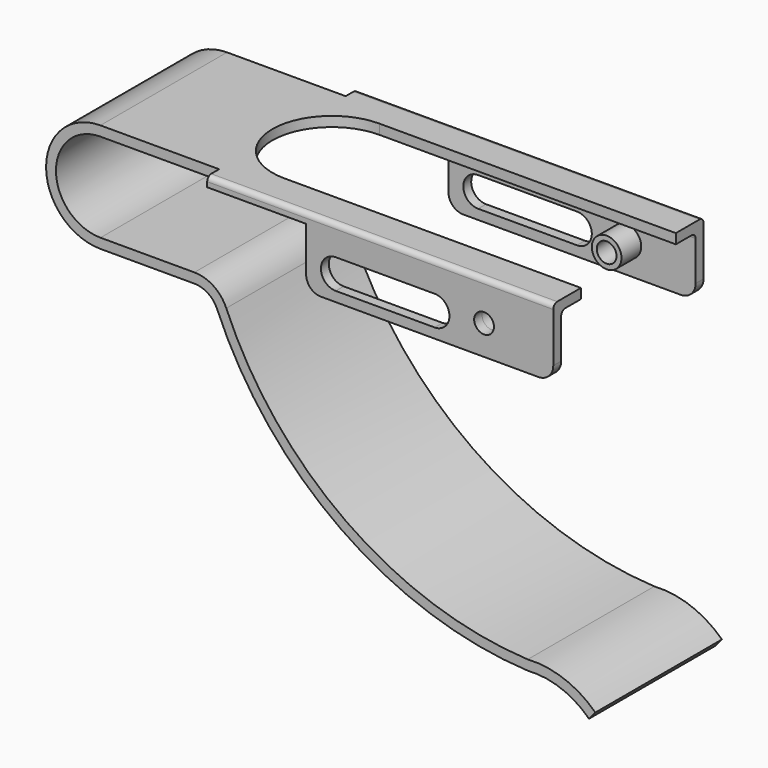
from build123d import *

# Parameters (mm, degrees)
F1_DEPTH  = 16
F2_W      = 70
F2_H      = 3
F3_DEPTH  = 2
F4_W      = 50
F4_H      = 12
F5_DEPTH  = 2
F6_R      = 1
F9_DEPTH  = 2
F11_DEPTH = 38.001
F13_D     = 4
F14_R     = 3
F14_R_2   = 2
F15_DEPTH = 5
F16_R     = 3


# Not quite as in the source:
# - a pattern or mirror of a feature is missing from the dataset's text; its kind, count and spacing are read off the source's solid


with BuildPart() as f1:
    # F0 (on Front) → F1 (new body)
    with BuildSketch(Plane.XZ):
        with BuildLine():
            Line((94, 11), (0, 11))
            ThreePointArc((0, 11), (-11, 0), (0, -11))
            Line((0, -11), (19, -11))
            ThreePointArc((19, -11), (21.7648271935, -11.8339790459), (23.607331209, -14.0577077639))
            ThreePointArc((23.607331209, -14.0577077639), (48.6917034204, -45.0930519948), (86.4506679072, -58.0034711071))
            ThreePointArc((86.4506679072, -58.0034711071), (93.1291053538, -58.9355091014), (98.8304523125, -62.5361846502))
            Line((98.8304523125, -62.5361846502), (100.1194642859, -61))
            ThreePointArc((100.1194642859, -61), (93.803453137, -57.0525770858), (86.4301074938, -56))
            ThreePointArc((86.4301074938, -56), (49.7895156694, -43.4202136678), (25.4502636926, -13.2807908695))
            ThreePointArc((25.4502636926, -13.2807908695), (22.8707580709, -10.1675706642), (19, -9))
            Line((19, -9), (0, -9))
            ThreePointArc((0, -9), (-9, 0), (0, 9))
            Line((0, 9), (94, 9))
            Line((94, 9), (94, 11))
        make_face()
    extrude(amount=F1_DEPTH)

    # F2 (on face) → F3 (join)
    with BuildSketch(Plane.XY.offset(11)):
        with Locations((59, -17.5)):
            Rectangle(F2_W, F2_H)
    extrude(amount=-F3_DEPTH)

    # F4 (on face) → F5 (join)
    with BuildSketch(Plane.XZ.offset(19)):
        with Locations((69, 3)):
            Rectangle(F4_W, F4_H)
    extrude(amount=-F5_DEPTH)

    # F6
    f6_edges = [f1.edges().sort_by_distance(p)[0] for p in [
        (59, -19, 11),
        (69, -17, 9),
    ]]
    fillet(f6_edges, radius=F6_R)

    # F7: F1 across plane


with BuildPart() as f1_1:
    add(f1.part)
    add(f1.part.mirror(Plane.XZ))

    # F8 (on face) → F9 (cut)
    with BuildSketch(Plane.XY.offset(11)):
        with BuildLine():
            Line((94, 12), (34, 12))
            ThreePointArc((34, 12), (22, 0), (34, -12))
            Line((34, -12), (94, -12))
            Line((94, -12), (94, 12))
        make_face()
    extrude(amount=-F9_DEPTH, mode=Mode.SUBTRACT)

    # F10 (on face) → F11 (cut, through all)
    with BuildSketch(Plane.XZ.offset(19)):
        with BuildLine():
            ThreePointArc((50, 5), (47, 2), (50, -1))
            Line((50, -1), (70, -1))
            ThreePointArc((70, -1), (73, 2), (70, 5))
            Line((70, 5), (50, 5))
        make_face()
    extrude(amount=-F11_DEPTH, mode=Mode.SUBTRACT)

    # F13 (through all)
    with Locations(Plane.XZ.offset(19)):
        with Locations((80, 3)):
            Hole(F13_D / 2)

    # F14 (on face) → F15 (join)
    with BuildSketch(Plane(origin=(0, -17, 0), x_dir=(-1, 0, 0), z_dir=(0, 1, 0))):
        with Locations((-80, 3)):
            Circle(F14_R)
        with Locations((-80, 3)):
            Circle(F14_R_2, mode=Mode.SUBTRACT)
    f15 = extrude(amount=F15_DEPTH)

    # F15_copies: F15 across plane
    add(f15.mirror(Plane.ZX))

    # F16
    f16_edges = [f1_1.edges().sort_by_distance(p)[0] for p in [
        (94, 18, -3),
        (44, 18, -3),
        (44, -18, -3),
        (94, -18, -3),
    ]]
    fillet(f16_edges, radius=F16_R)


solid = f1_1.part
